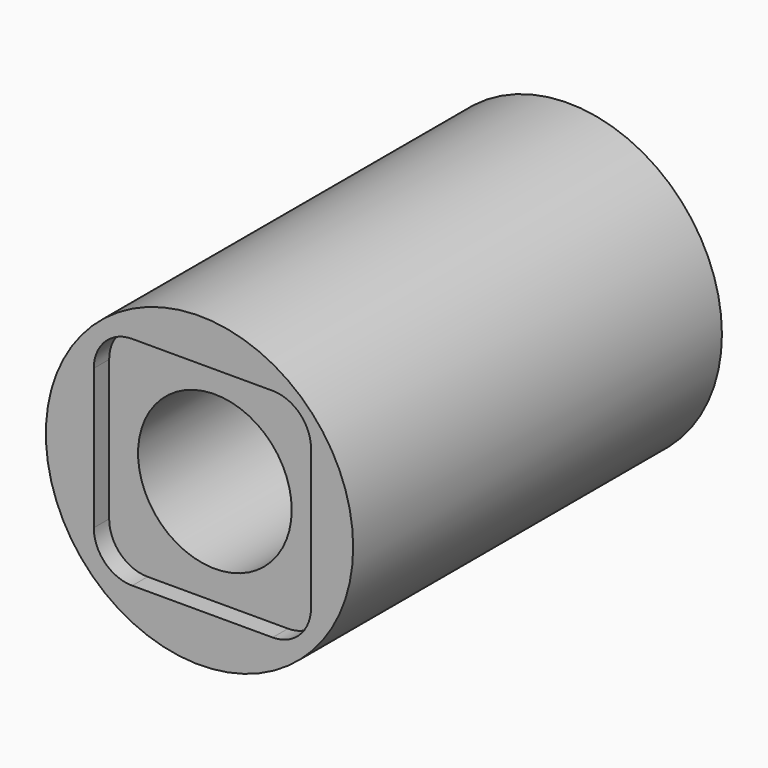
from build123d import *

# Parameters (mm, degrees)
F0_R          = 4
F0_R_2        = 2
F1_DEPTH      = 6
F1_DEPTH_BACK = 6
F2_R          = 2
F3_DEPTH      = 0.5


# Not quite as in the source:
# - a pattern or mirror of a feature is missing from the dataset's text; its kind, count and spacing are read off the source's solid


with BuildPart() as f1:
    # F0 (on Front) → F1 (new body, two sides)
    with BuildSketch(Plane.XZ) as f1_sk:
        Circle(F0_R)
        Circle(F0_R_2, mode=Mode.SUBTRACT)
    extrude(amount=F1_DEPTH)
    extrude(f1_sk.sketch, amount=-F1_DEPTH_BACK)

    # F2 (on face) → F3 (cut)
    with BuildSketch(Plane.XZ.offset(6)):
        with BuildLine():
            Line((1.902670174, 2.902670174), (-1.7521820182, 2.902670174))
            ThreePointArc((-1.7521820182, 2.902670174), (-2.4592887994, 2.6097769551), (-2.7521820182, 1.902670174))
            Line((-2.7521820182, 1.902670174), (-2.7521820182, -1.7521820182))
            ThreePointArc((-2.7521820182, -1.7521820182), (-2.4592887994, -2.4592887994), (-1.7521820182, -2.7521820182))
            Line((-1.7521820182, -2.7521820182), (1.902670174, -2.7521820182))
            ThreePointArc((1.902670174, -2.7521820182), (2.6097769551, -2.4592887994), (2.902670174, -1.7521820182))
            Line((2.902670174, -1.7521820182), (2.902670174, 1.902670174))
            ThreePointArc((2.902670174, 1.902670174), (2.6097769551, 2.6097769551), (1.902670174, 2.902670174))
        make_face()
        Circle(F2_R, mode=Mode.SUBTRACT)
    f3 = extrude(amount=-F3_DEPTH, mode=Mode.SUBTRACT)

    # F3_copies: F3 across plane
    add(f3.mirror(Plane.ZX), mode=Mode.SUBTRACT)


solid = f1.part
